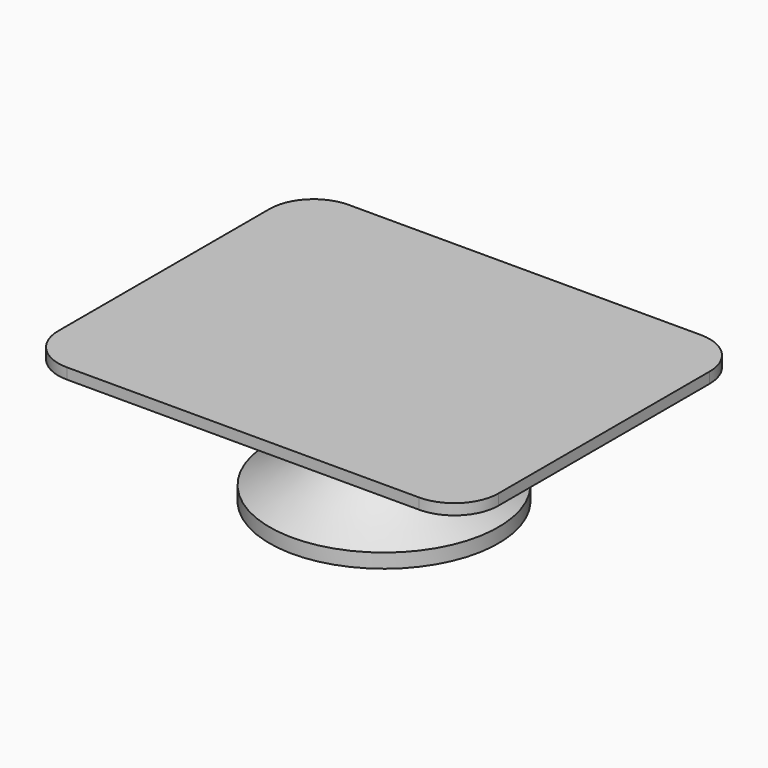
from build123d import *

# Parameters (mm, degrees)
F1_DEPTH     = 20
F2_DEPTH     = 13
F0_W         = 13
F0_H         = 1.6210880779
F4_T4_DEPTH  = 25
F4_T9_DEPTH  = 26
F4_T14_DEPTH = 26
F4_T19_DEPTH = 25
F4_T25_DEPTH = 38.8584149398
F4_T30_DEPTH = 37.8584149398
F4_T38_DEPTH = 37.8584149398
F4_T43_DEPTH = 38.8584149398
F4_T51_DEPTH = 38.8584149398
F4_T56_DEPTH = 37.8584149398
F4_T64_DEPTH = 38.8584149398
F4_T69_DEPTH = 37.8584149398
F5_R         = 5
F6_R         = 5


# Not quite as in the source:
# - a fillet or chamfer that OpenCascade refuses, or shapes differently, is made with other operations: its cross-section is extruded or revolved along the edge and cut away or added


with BuildPart() as f1:
    # F0 (on Front) → F1 (new body, symmetric)
    with BuildSketch(Plane.XZ):
        Polygon((0, 13.7715186066), (0, 15), (-25, 15), (-25, 13.7715186066), (-12.5, 13.7715186066), align=None)
        Polygon((25, 15), (0, 15), (0, 13.7715186066), (12.5, 13.7715186066), (25, 13.7715186066), align=None)
    extrude(amount=F1_DEPTH, both=True)

    # F0 (on Front) → F2 (join, symmetric)
    with BuildSketch(Plane.XZ):
        Polygon((0, 12.6210880779), (0, 13.7715186066), (-12.5, 13.7715186066), (-12.5, 12.6210880779), (-6.25, 12.6210880779), align=None)
        Polygon((12.5, 13.7715186066), (0, 13.7715186066), (0, 12.6210880779), (6.25, 12.6210880779), (12.5, 12.6210880779), align=None)
    extrude(amount=F2_DEPTH, both=True)

    # F4: chamfer of 5 on 4 edges, made by hand


with BuildPart() as f2:
    # F0 (on Front) → F2, piece 2 (new body, symmetric)
    with BuildSketch(Plane.XZ):
        with Locations((-6.5, 0.810544039)):
            Rectangle(F0_W, F0_H)
        with Locations((6.5, 0.810544039)):
            Rectangle(F0_W, F0_H)
    extrude(amount=F2_DEPTH, both=True)

    # F5
    f5_edges = [f2.edges().sort_by_distance(p)[0] for p in [
        (-13, 13, 0.810544),
        (-13, -13, 0.810544),
        (13, -13, 0.810544),
        (13, 13, 0.810544),
    ]]
    fillet(f5_edges, radius=F5_R)


with BuildPart() as f3:
    # F0 (on Front) → F3 (revolve)
    with BuildSketch(Plane.XZ):
        with BuildLine():
            Line((0, 1.6210880779), (0, 12.6210880779))
            Line((0, 12.6210880779), (-6.25, 12.6210880779))
            add(Edge.make_bspline(
                [(-13, 1.6210880779), (-4.3921764009, 6.5395440906), (-6.2563242824, 10.3996003671), (-6.25, 12.6210880779)],
                knots=[0, 0, 0, 0, 12.9059094991, 12.9059094991, 12.9059094991, 12.9059094991], degree=3))
            Line((-13, 1.6210880779), (0, 1.6210880779))
        make_face()
    revolve(axis=Axis((0, 0, 7.5), (0, 0, -1)))

    # F0 (on Front) → F8 (revolve)
    with BuildSketch(Plane.XZ):
        with Locations((-6.5, 0.810544039)):
            Rectangle(F0_W, F0_H)
    revolve(axis=Axis((0, 0, 0.810544039), (0, 0, -1)))


with BuildPart() as f4_tool2:
    # F4_s3 → F4_t4 (new body)
    with BuildSketch(Plane.YZ.offset(-12.5)):
        with BuildLine():
            Line((13.1414213562, 17.7625094341), (7.8585786438, 12.4796667217))
            Line((7.8585786438, 12.4796667217), (7.8585786438, 12.3796667217))
            ThreePointArc((7.8585786438, 12.3796667217), (10.4292893219, 12.5210880779), (13, 12.5210880779))
            Line((13, 12.5210880779), (13.1, 12.6210880779))
            ThreePointArc((13.1, 12.6210880779), (13.1, 15.191798756), (13.2414213562, 17.7625094341))
            Line((13.2414213562, 17.7625094341), (13.1414213562, 17.7625094341))
        make_face()
    extrude(amount=F4_T4_DEPTH)

    split(bisect_by=Plane.XY.offset(13.7715186066), keep=Keep.BOTTOM)


with BuildPart() as f1_1:
    add(f1.part)

    # F4_t1: cut F4_tool2
    add(f4_tool2.part, mode=Mode.SUBTRACT)


with BuildPart() as f4_tool7:
    # F4_s8 → F4_t9 (new body)
    with BuildSketch(Plane.XZ.offset(-13)):
        with BuildLine():
            Line((-12.6414213562, 17.7625094341), (-7.3585786438, 12.4796667217))
            Line((-7.3585786438, 12.4796667217), (-7.3585786438, 12.3796667217))
            ThreePointArc((-7.3585786438, 12.3796667217), (-9.9292893219, 12.5210880779), (-12.5, 12.5210880779))
            Line((-12.5, 12.5210880779), (-12.6, 12.6210880779))
            ThreePointArc((-12.6, 12.6210880779), (-12.6, 15.191798756), (-12.7414213562, 17.7625094341))
            Line((-12.7414213562, 17.7625094341), (-12.6414213562, 17.7625094341))
        make_face()
    extrude(amount=F4_T9_DEPTH)

    split(bisect_by=Plane.XY.offset(13.7715186066), keep=Keep.BOTTOM)


with BuildPart() as f1_2:
    add(f1_1.part)

    # F4_t6: cut F4_tool7
    add(f4_tool7.part, mode=Mode.SUBTRACT)


with BuildPart() as f4_tool12:
    # F4_s13 → F4_t14 (new body)
    with BuildSketch(Plane.XZ.offset(-13)):
        with BuildLine():
            Line((12.6414213562, 17.7625094341), (7.3585786438, 12.4796667217))
            Line((7.3585786438, 12.4796667217), (7.3585786438, 12.3796667217))
            ThreePointArc((7.3585786438, 12.3796667217), (9.9292893219, 12.5210880779), (12.5, 12.5210880779))
            Line((12.5, 12.5210880779), (12.6, 12.6210880779))
            ThreePointArc((12.6, 12.6210880779), (12.6, 15.191798756), (12.7414213562, 17.7625094341))
            Line((12.7414213562, 17.7625094341), (12.6414213562, 17.7625094341))
        make_face()
    extrude(amount=F4_T14_DEPTH)

    split(bisect_by=Plane.XY.offset(13.7715186066), keep=Keep.BOTTOM)


with BuildPart() as f1_3:
    add(f1_2.part)

    # F4_t11: cut F4_tool12
    add(f4_tool12.part, mode=Mode.SUBTRACT)


with BuildPart() as f4_tool17:
    # F4_s18 → F4_t19 (new body)
    with BuildSketch(Plane.YZ.offset(-12.5)):
        with BuildLine():
            Line((-13.1414213562, 17.7625094341), (-7.8585786438, 12.4796667217))
            Line((-7.8585786438, 12.4796667217), (-7.8585786438, 12.3796667217))
            ThreePointArc((-7.8585786438, 12.3796667217), (-10.4292893219, 12.5210880779), (-13, 12.5210880779))
            Line((-13, 12.5210880779), (-13.1, 12.6210880779))
            ThreePointArc((-13.1, 12.6210880779), (-13.1, 15.191798756), (-13.2414213562, 17.7625094341))
            Line((-13.2414213562, 17.7625094341), (-13.1414213562, 17.7625094341))
        make_face()
    extrude(amount=F4_T19_DEPTH)

    split(bisect_by=Plane.XY.offset(13.7715186066), keep=Keep.BOTTOM)


with BuildPart() as f1_4:
    add(f1_3.part)

    # F4_t16: cut F4_tool17
    add(f4_tool17.part, mode=Mode.SUBTRACT)


with BuildPart() as f4_tool23:
    # F4_s24 → F4_t25 (new body)
    with BuildSketch(Plane.XZ.offset(-25.8584149398)):
        with BuildLine():
            Line((-12.6414213562, 17.7625094341), (-7.3585786438, 12.4796667217))
            Line((-7.3585786438, 12.4796667217), (-7.3585786438, 12.3796667217))
            ThreePointArc((-7.3585786438, 12.3796667217), (-9.9292893219, 12.5210880779), (-12.5, 12.5210880779))
            Line((-12.5, 12.5210880779), (-12.6, 12.6210880779))
            ThreePointArc((-12.6, 12.6210880779), (-12.6, 15.191798756), (-12.7414213562, 17.7625094341))
            Line((-12.7414213562, 17.7625094341), (-12.6414213562, 17.7625094341))
        make_face()
    extrude(amount=F4_T25_DEPTH)

    split(bisect_by=Plane.XY.offset(13.7715186066), keep=Keep.BOTTOM)

    split(bisect_by=Plane.XZ.offset(-13), keep=Keep.BOTTOM)


with BuildPart() as f4_tool28:
    # F4_s29 → F4_t30 (new body)
    with BuildSketch(Plane.YZ.offset(-25.3584149398)):
        with BuildLine():
            Line((13.1414213562, 17.7625094341), (7.8585786438, 12.4796667217))
            Line((7.8585786438, 12.4796667217), (7.8585786438, 12.3796667217))
            ThreePointArc((7.8585786438, 12.3796667217), (10.4292893219, 12.5210880779), (13, 12.5210880779))
            Line((13, 12.5210880779), (13.1, 12.6210880779))
            ThreePointArc((13.1, 12.6210880779), (13.1, 15.191798756), (13.2414213562, 17.7625094341))
            Line((13.2414213562, 17.7625094341), (13.1414213562, 17.7625094341))
        make_face()
    extrude(amount=F4_T30_DEPTH)

    split(bisect_by=Plane.XY.offset(13.7715186066), keep=Keep.BOTTOM)

    split(bisect_by=Plane.YZ.offset(-12.5), keep=Keep.BOTTOM)


with BuildPart() as f4_tool23_1:
    add(f4_tool23.part)

    # F4_t33: intersect F4_tool28
    add(f4_tool28.part, mode=Mode.INTERSECT)


with BuildPart() as f1_5:
    add(f1_4.part)

    # F4_t21: cut F4_tool23
    add(f4_tool23_1.part, mode=Mode.SUBTRACT)


with BuildPart() as f4_tool36:
    # F4_s37 → F4_t38 (new body)
    with BuildSketch(Plane.YZ.offset(-12.5)):
        with BuildLine():
            Line((13.1414213562, 17.7625094341), (7.8585786438, 12.4796667217))
            Line((7.8585786438, 12.4796667217), (7.8585786438, 12.3796667217))
            ThreePointArc((7.8585786438, 12.3796667217), (10.4292893219, 12.5210880779), (13, 12.5210880779))
            Line((13, 12.5210880779), (13.1, 12.6210880779))
            ThreePointArc((13.1, 12.6210880779), (13.1, 15.191798756), (13.2414213562, 17.7625094341))
            Line((13.2414213562, 17.7625094341), (13.1414213562, 17.7625094341))
        make_face()
    extrude(amount=F4_T38_DEPTH)

    split(bisect_by=Plane.XY.offset(13.7715186066), keep=Keep.BOTTOM)

    split(bisect_by=Plane.YZ.offset(12.5), keep=Keep.TOP)


with BuildPart() as f4_tool41:
    # F4_s42 → F4_t43 (new body)
    with BuildSketch(Plane.XZ.offset(-25.8584149398)):
        with BuildLine():
            Line((12.6414213562, 17.7625094341), (7.3585786438, 12.4796667217))
            Line((7.3585786438, 12.4796667217), (7.3585786438, 12.3796667217))
            ThreePointArc((7.3585786438, 12.3796667217), (9.9292893219, 12.5210880779), (12.5, 12.5210880779))
            Line((12.5, 12.5210880779), (12.6, 12.6210880779))
            ThreePointArc((12.6, 12.6210880779), (12.6, 15.191798756), (12.7414213562, 17.7625094341))
            Line((12.7414213562, 17.7625094341), (12.6414213562, 17.7625094341))
        make_face()
    extrude(amount=F4_T43_DEPTH)

    split(bisect_by=Plane.XY.offset(13.7715186066), keep=Keep.BOTTOM)

    split(bisect_by=Plane.XZ.offset(-13), keep=Keep.BOTTOM)


with BuildPart() as f4_tool36_1:
    add(f4_tool36.part)

    # F4_t46: intersect F4_tool41
    add(f4_tool41.part, mode=Mode.INTERSECT)


with BuildPart() as f1_6:
    add(f1_5.part)

    # F4_t34: cut F4_tool36
    add(f4_tool36_1.part, mode=Mode.SUBTRACT)


with BuildPart() as f4_tool49:
    # F4_s50 → F4_t51 (new body)
    with BuildSketch(Plane.XZ.offset(-13)):
        with BuildLine():
            Line((-12.6414213562, 17.7625094341), (-7.3585786438, 12.4796667217))
            Line((-7.3585786438, 12.4796667217), (-7.3585786438, 12.3796667217))
            ThreePointArc((-7.3585786438, 12.3796667217), (-9.9292893219, 12.5210880779), (-12.5, 12.5210880779))
            Line((-12.5, 12.5210880779), (-12.6, 12.6210880779))
            ThreePointArc((-12.6, 12.6210880779), (-12.6, 15.191798756), (-12.7414213562, 17.7625094341))
            Line((-12.7414213562, 17.7625094341), (-12.6414213562, 17.7625094341))
        make_face()
    extrude(amount=F4_T51_DEPTH)

    split(bisect_by=Plane.XY.offset(13.7715186066), keep=Keep.BOTTOM)

    split(bisect_by=Plane.XZ.offset(13), keep=Keep.TOP)


with BuildPart() as f4_tool54:
    # F4_s55 → F4_t56 (new body)
    with BuildSketch(Plane.YZ.offset(-25.3584149398)):
        with BuildLine():
            Line((-13.1414213562, 17.7625094341), (-7.8585786438, 12.4796667217))
            Line((-7.8585786438, 12.4796667217), (-7.8585786438, 12.3796667217))
            ThreePointArc((-7.8585786438, 12.3796667217), (-10.4292893219, 12.5210880779), (-13, 12.5210880779))
            Line((-13, 12.5210880779), (-13.1, 12.6210880779))
            ThreePointArc((-13.1, 12.6210880779), (-13.1, 15.191798756), (-13.2414213562, 17.7625094341))
            Line((-13.2414213562, 17.7625094341), (-13.1414213562, 17.7625094341))
        make_face()
    extrude(amount=F4_T56_DEPTH)

    split(bisect_by=Plane.XY.offset(13.7715186066), keep=Keep.BOTTOM)

    split(bisect_by=Plane.YZ.offset(-12.5), keep=Keep.BOTTOM)


with BuildPart() as f4_tool49_1:
    add(f4_tool49.part)

    # F4_t59: intersect F4_tool54
    add(f4_tool54.part, mode=Mode.INTERSECT)


with BuildPart() as f1_7:
    add(f1_6.part)

    # F4_t47: cut F4_tool49
    add(f4_tool49_1.part, mode=Mode.SUBTRACT)


with BuildPart() as f4_tool62:
    # F4_s63 → F4_t64 (new body)
    with BuildSketch(Plane.XZ.offset(-13)):
        with BuildLine():
            Line((12.6414213562, 17.7625094341), (7.3585786438, 12.4796667217))
            Line((7.3585786438, 12.4796667217), (7.3585786438, 12.3796667217))
            ThreePointArc((7.3585786438, 12.3796667217), (9.9292893219, 12.5210880779), (12.5, 12.5210880779))
            Line((12.5, 12.5210880779), (12.6, 12.6210880779))
            ThreePointArc((12.6, 12.6210880779), (12.6, 15.191798756), (12.7414213562, 17.7625094341))
            Line((12.7414213562, 17.7625094341), (12.6414213562, 17.7625094341))
        make_face()
    extrude(amount=F4_T64_DEPTH)

    split(bisect_by=Plane.XY.offset(13.7715186066), keep=Keep.BOTTOM)

    split(bisect_by=Plane.XZ.offset(13), keep=Keep.TOP)


with BuildPart() as f4_tool67:
    # F4_s68 → F4_t69 (new body)
    with BuildSketch(Plane.YZ.offset(-12.5)):
        with BuildLine():
            Line((-13.1414213562, 17.7625094341), (-7.8585786438, 12.4796667217))
            Line((-7.8585786438, 12.4796667217), (-7.8585786438, 12.3796667217))
            ThreePointArc((-7.8585786438, 12.3796667217), (-10.4292893219, 12.5210880779), (-13, 12.5210880779))
            Line((-13, 12.5210880779), (-13.1, 12.6210880779))
            ThreePointArc((-13.1, 12.6210880779), (-13.1, 15.191798756), (-13.2414213562, 17.7625094341))
            Line((-13.2414213562, 17.7625094341), (-13.1414213562, 17.7625094341))
        make_face()
    extrude(amount=F4_T69_DEPTH)

    split(bisect_by=Plane.XY.offset(13.7715186066), keep=Keep.BOTTOM)

    split(bisect_by=Plane.YZ.offset(12.5), keep=Keep.TOP)


with BuildPart() as f4_tool62_1:
    add(f4_tool62.part)

    # F4_t72: intersect F4_tool67
    add(f4_tool67.part, mode=Mode.INTERSECT)


with BuildPart() as f1_8:
    add(f1_7.part)

    # F4_t60: cut F4_tool62
    add(f4_tool62_1.part, mode=Mode.SUBTRACT)

    # F6
    f6_edges = [f1_8.edges().sort_by_distance(p)[0] for p in [
        (-25, -20, 14.385759),
        (-25, 20, 14.385759),
        (25, -20, 14.385759),
        (25, 20, 14.385759),
    ]]
    fillet(f6_edges, radius=F6_R)


solid = Compound([f3.part, f1_8.part])
